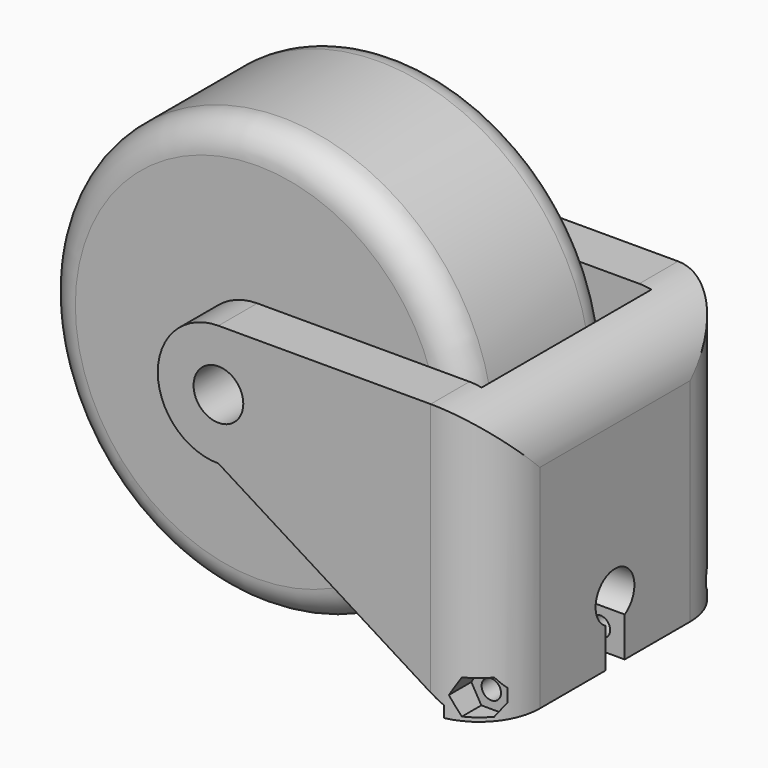
from build123d import *

# Parameters (mm, degrees)
F0_R         = 35
F0_R_2       = 4
F1_DEPTH     = 30
F2_R         = 5
F3_R         = 4.1
F4_DEPTH     = 8
F7_W         = 51
F7_H         = 45
F8_DEPTH     = 8
F11_DEPTH    = 8
F12_R        = 1.6
F13_DEPTH    = 51
F14_R        = 2.85
F15_DEPTH    = 15
F17_DEPTH    = 5
F18_T1_DEPTH = 58
F18_T3_DEPTH = 58
F18_T5_DEPTH = 101
F18_T7_DEPTH = 95


# Not quite as in the source:
# - a fillet or chamfer that OpenCascade refuses, or shapes differently, is made with other operations: its cross-section is extruded or revolved along the edge and cut away or added


with BuildPart() as f1:
    # F0 (on Front) → F1 (new body)
    with BuildSketch(Plane.XZ):
        Circle(F0_R)
        Circle(F0_R_2, mode=Mode.SUBTRACT)
    extrude(amount=F1_DEPTH)

    # F2
    f2_edges = [f1.edges().sort_by_distance(p)[0] for p in [
        (-35, -30, 0),
        (-35, 0, 0),
    ]]
    fillet(f2_edges, radius=F2_R)


with BuildPart() as f4:
    # F3 (on face) → F4 (new body)
    with BuildSketch(Plane.XZ.offset(30)):
        Polygon((45, 10), (0, 10), (-10, 10), (-10, -10), (0, -10), (40, -35), (45, -35), align=None)
        Circle(F3_R, mode=Mode.SUBTRACT)
    extrude(amount=F4_DEPTH)


with BuildPart() as f5_1:
    # F5: instance of F4
    add(f4.part.mirror(Plane(origin=(22.6623991549, -30, -7.1637600407), x_dir=(-1, 0, 0), z_dir=(0, 1, 0))))


with BuildPart() as f5_1_1:
    # F6: moved
    add(f5_1.part.moved(Location((0, 35, 0))))


with BuildPart() as f8:
    # F7 (on face) → F8 (new body)
    with BuildSketch(Plane.YZ.offset(45)):
        with Locations((-12.5, -12.5)):
            Rectangle(F7_W, F7_H)
    extrude(amount=-F8_DEPTH)


with BuildPart() as f4_1:
    add(f4.part)

    # F9: union F8, F5_1
    add(f8.part)
    add(f5_1_1.part)

    # F10 (on face) → F11 (cut)
    with BuildSketch(Plane.YZ.offset(45)):
        with BuildLine():
            Line((-14.5, -35), (-12.5, -35))
            Line((-12.5, -35), (-10.5, -35))
            Line((-10.5, -35), (-10.5, -28.4641016151))
            ThreePointArc((-10.5, -28.4641016151), (-12.5, -21), (-14.5, -28.4641016151))
            Line((-14.5, -28.4641016151), (-14.5, -35))
        make_face()
    extrude(amount=-F11_DEPTH, mode=Mode.SUBTRACT)

    # F12 (on face) → F13 (cut)
    with BuildSketch(Plane(origin=(0, 13, 0), x_dir=(-1, 0, 0), z_dir=(0, 1, 0))):
        with Locations((-41, -31.5)):
            Circle(F12_R)
    extrude(amount=-F13_DEPTH, mode=Mode.SUBTRACT)

    # F14 (on face) → F15 (cut)
    with BuildSketch(Plane(origin=(0, 13, 0), x_dir=(-1, 0, 0), z_dir=(0, 1, 0))):
        with Locations((-41, -31.5)):
            Circle(F14_R)
    extrude(amount=-F15_DEPTH, mode=Mode.SUBTRACT)

    # F16 (on face) → F17 (cut)
    with BuildSketch(Plane.XZ.offset(38)):
        Polygon((42.6454482672, -28.65), (39.3545517328, -28.65), (37.7091034656, -31.5), (39.3545517328, -34.35), (42.6454482672, -34.35), (44.2908965344, -31.5), align=None)
    extrude(amount=-F17_DEPTH, mode=Mode.SUBTRACT)

    # F18: fillet of radius 10 on 7 edges, made by hand

    # F18_s2 → F18_t1 (cut)
    with BuildSketch(Plane.XZ.offset(5)):
        with BuildLine():
            ThreePointArc((-10, 0), (-7.0710678119, -7.0710678119), (0, -10))
            Line((0, -10), (-10, -10))
            Line((-10, -10), (-10, 0))
        make_face()
        with BuildLine():
            ThreePointArc((0, 10), (-7.0710678119, 7.0710678119), (-10, 0))
            Line((-10, 0), (-10, 10))
            Line((-10, 10), (0, 10))
        make_face()
    extrude(amount=F18_T1_DEPTH, mode=Mode.SUBTRACT)

    # F18_s4 → F18_t3 (cut)
    with BuildSketch(Plane.XZ.offset(-38)):
        with BuildLine():
            ThreePointArc((-10, 0), (-7.0710678119, -7.0710678119), (0, -10))
            Line((0, -10), (-10, -10))
            Line((-10, -10), (-10, 0))
        make_face()
        with BuildLine():
            ThreePointArc((0, 10), (-7.0710678119, 7.0710678119), (-10, 0))
            Line((-10, 0), (-10, 10))
            Line((-10, 10), (0, 10))
        make_face()
    extrude(amount=F18_T3_DEPTH, mode=Mode.SUBTRACT)

    # F18_s6 → F18_t5 (cut)
    with BuildSketch(Plane.XZ.offset(-38)):
        with BuildLine():
            ThreePointArc((35, 10), (42.0710678119, 7.0710678119), (45, 0))
            Line((45, 0), (45, 10))
            Line((45, 10), (35, 10))
        make_face()
    extrude(amount=F18_T5_DEPTH, mode=Mode.SUBTRACT)

    # F18_s8 → F18_t7 (cut)
    with BuildSketch(Plane.XY.offset(-60)):
        with BuildLine():
            ThreePointArc((35, 13), (42.0710678119, 10.0710678119), (45, 3))
            Line((45, 3), (45, 13))
            Line((45, 13), (35, 13))
        make_face()
        with BuildLine():
            ThreePointArc((35, -38), (42.0710678119, -35.0710678119), (45, -28))
            Line((45, -28), (45, -38))
            Line((45, -38), (35, -38))
        make_face()
    extrude(amount=F18_T7_DEPTH, mode=Mode.SUBTRACT)


solid = Compound([f1.part, f4_1.part])
